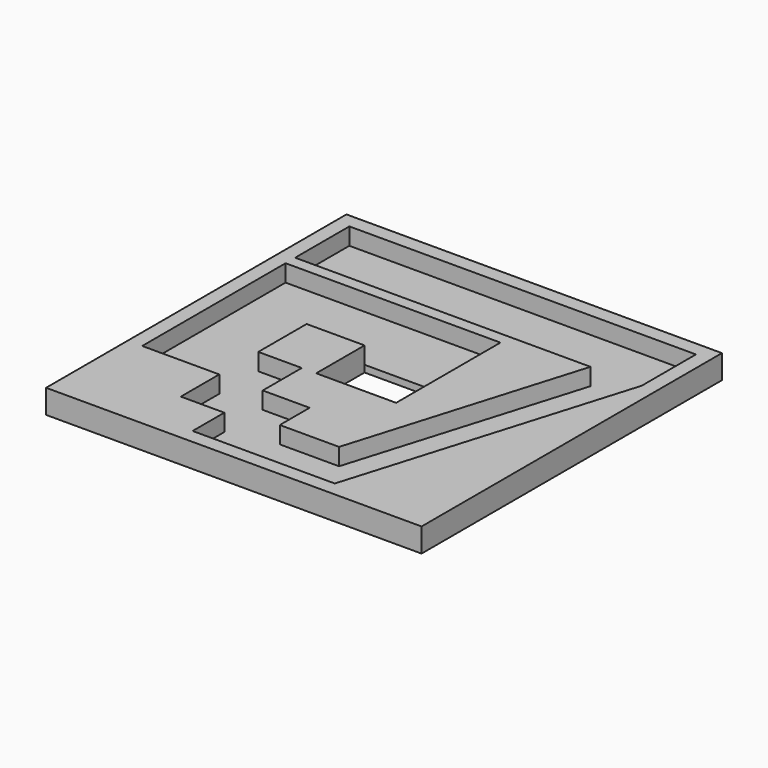
from build123d import *

# Parameters (mm, degrees)
F1_DEPTH = 5
F2_DEPTH = 2


# Not quite as in the source:
# - a feature names something its author has since deleted; it is built from what else it names


with BuildPart() as f1:
    # F0 (on Top) → F1 (new body)
    with BuildSketch(Plane.XY):
        Polygon((-53.2781591106, 53.5204063327), (-53.2781591106, -56.4795936673), (-13.7344817631, -56.4795936673), (56.7218408894, -56.4795936673), (56.7218408894, 53.5204063327), align=None)
        Polygon((-49.0473898798, 29.4351325184), (-49.0473898798, 49.289637102), (52.4910716586, 49.289637102), (52.4910716586, 29.4351325184), (27.9224817305, -52.2488244365), (-13.7344817631, -52.2488244365), (-13.7344817631, -40.6398742527), (-26.4708319562, -40.6398742527), (-26.4708319562, -26.5670741801), (-49.0473898798, -26.5670741801), (-49.0473898798, 5.428542512), (-49.0473898798, 25.9305896417), (-26.4708319562, 25.9305896417), (13.9133328608, 25.9305896417), (13.9133328608, 5.428542512), (13.9133328608, -12.2777693511), (-9.5037125323, -12.2777693511), (-9.5037125323, 5.428542512), (-26.4708319562, 5.428542512), (-26.4708319562, -12.2777693511), (-13.7344817631, -12.2777693511), (-13.7344817631, -26.5670741801), (0, -26.5670741801), (0, -37.4845501322), (17.3598656954, -37.4845501322), (37.487713347, 29.4351325184), align=None, mode=Mode.SUBTRACT)
    extrude(amount=F1_DEPTH)

    # F0 (on Top) → F2 (join)
    with BuildSketch(Plane.XY):
        Polygon((-53.2781591106, 53.5204063327), (-53.2781591106, -56.4795936673), (-13.7344817631, -56.4795936673), (56.7218408894, -56.4795936673), (56.7218408894, 53.5204063327), align=None)
        Polygon((-49.0473898798, 29.4351325184), (-49.0473898798, 49.289637102), (52.4910716586, 49.289637102), (52.4910716586, 29.4351325184), (27.9224817305, -52.2488244365), (-13.7344817631, -52.2488244365), (-13.7344817631, -40.6398742527), (-26.4708319562, -40.6398742527), (-26.4708319562, -26.5670741801), (-49.0473898798, -26.5670741801), (-49.0473898798, 5.428542512), (-49.0473898798, 25.9305896417), (-26.4708319562, 25.9305896417), (13.9133328608, 25.9305896417), (13.9133328608, 5.428542512), (13.9133328608, -12.2777693511), (-9.5037125323, -12.2777693511), (-9.5037125323, 5.428542512), (-26.4708319562, 5.428542512), (-26.4708319562, -12.2777693511), (-13.7344817631, -12.2777693511), (-13.7344817631, -26.5670741801), (0, -26.5670741801), (0, -37.4845501322), (17.3598656954, -37.4845501322), (37.487713347, 29.4351325184), align=None, mode=Mode.SUBTRACT)
        Polygon((52.4910716586, 49.289637102), (-49.0473898798, 49.289637102), (-49.0473898798, 29.4351325184), (37.487713347, 29.4351325184), (17.3598656954, -37.4845501322), (0, -37.4845501322), (0, -26.5670741801), (-13.7344817631, -26.5670741801), (-13.7344817631, -12.2777693511), (-26.4708319562, -12.2777693511), (-26.4708319562, 5.428542512), (-9.5037125323, 5.428542512), (13.9133328608, 5.428542512), (13.9133328608, 25.9305896417), (-26.4708319562, 25.9305896417), (-49.0473898798, 25.9305896417), (-49.0473898798, 5.428542512), (-49.0473898798, -26.5670741801), (-26.4708319562, -26.5670741801), (-26.4708319562, -40.6398742527), (-13.7344817631, -40.6398742527), (-13.7344817631, -52.2488244365), (27.9224817305, -52.2488244365), (52.4910716586, 29.4351325184), align=None)
    extrude(amount=-F2_DEPTH)


solid = f1.part
